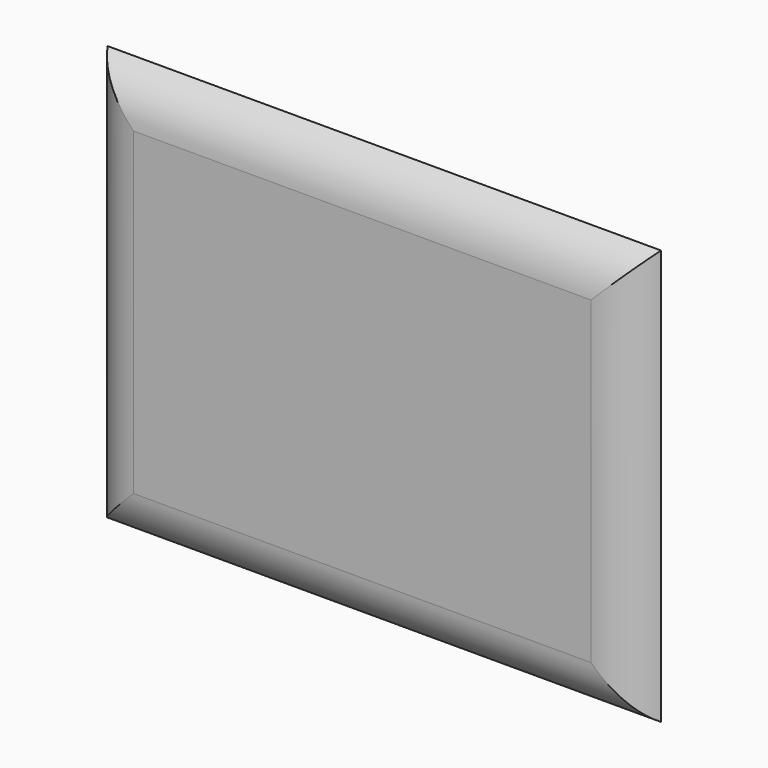
from build123d import *

# Parameters (mm, degrees)
F0_W        = 20
F0_H        = 15
F1_DEPTH    = 1
F2_T1_DEPTH = 28.6602540378
F2_T3_DEPTH = 23.6602540378
F3_W        = 16.5358983849
F3_H        = 11.5358983849
F4_DEPTH    = 1


# Not quite as in the source:
# - a fillet or chamfer that OpenCascade refuses, or shapes differently, is made with other operations: its cross-section is extruded or revolved along the edge and cut away or added


with BuildPart() as f1:
    # F0 (on Front) → F1 (new body)
    with BuildSketch(Plane.XZ):
        with Locations((2.3798597425, 3.1954329461)):
            Rectangle(F0_W, F0_H)
    extrude(amount=F1_DEPTH)

    # F2: fillet of radius 2 on 4 edges, made by hand

    # F2_s2 → F2_t1 (cut)
    with BuildSketch(Plane.YZ.offset(-11.9502672764)):
        with BuildLine():
            ThreePointArc((0, 10.6954329461), (-0.7320508076, 9.9633821385), (-1, 8.9633821385))
            Line((-1, 8.9633821385), (-1, 10.6954329461))
            Line((-1, 10.6954329461), (0, 10.6954329461))
        make_face()
        with BuildLine():
            ThreePointArc((0, -4.3045670539), (-0.7320508076, -3.5725162463), (-1, -2.5725162463))
            Line((-1, -2.5725162463), (-1, -4.3045670539))
            Line((-1, -4.3045670539), (0, -4.3045670539))
        make_face()
    extrude(amount=F2_T1_DEPTH, mode=Mode.SUBTRACT)

    # F2_s4 → F2_t3 (cut)
    with BuildSketch(Plane.XY.offset(-8.6346940728)):
        with BuildLine():
            ThreePointArc((12.3798597425, 0), (11.6478089349, -0.7320508076), (10.6478089349, -1))
            Line((10.6478089349, -1), (12.3798597425, -1))
            Line((12.3798597425, -1), (12.3798597425, 0))
        make_face()
        with BuildLine():
            ThreePointArc((-7.6201402575, 0), (-6.8880894499, -0.7320508076), (-5.8880894499, -1))
            Line((-5.8880894499, -1), (-7.6201402575, -1))
            Line((-7.6201402575, -1), (-7.6201402575, 0))
        make_face()
    extrude(amount=F2_T3_DEPTH, mode=Mode.SUBTRACT)


with BuildPart() as f4:
    # F3 (on face) → F4 (new body)
    with BuildSketch(Plane.XZ.offset(1)):
        with Locations((2.3798597425, 3.1954329461)):
            Rectangle(F3_W, F3_H)
    extrude(amount=-F4_DEPTH)


solid = Compound([f1.part, f4.part])
